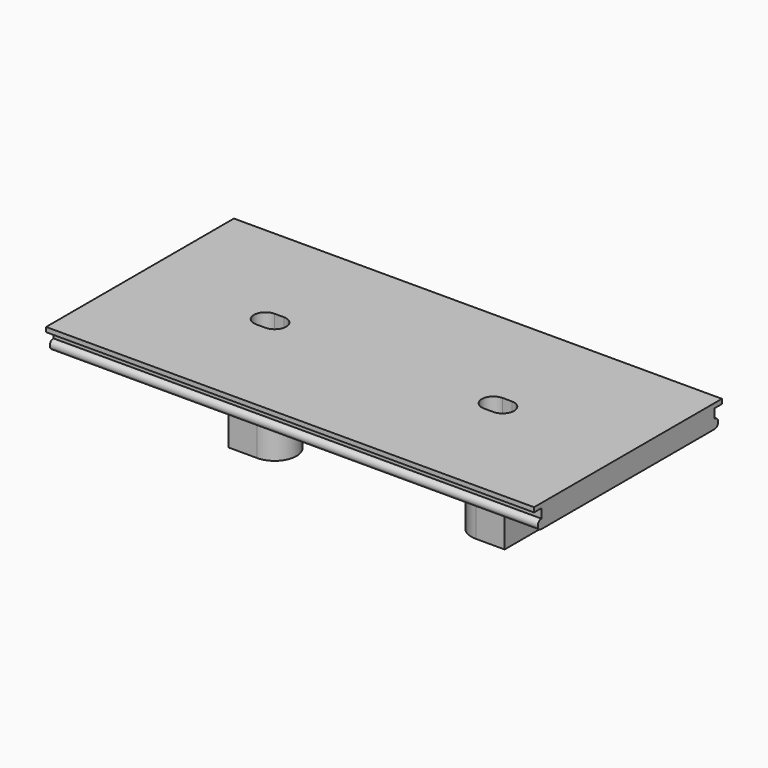
from build123d import *

# Parameters (mm, degrees)
F0_W     = 106
F0_H     = 47
F1_DEPTH = 2
F3_DEPTH = 1
F5_DEPTH = 106
F7_DEPTH = 19
F8_DEPTH = 25


with BuildPart() as f1:
    # F0 (on Top) → F1 (new body)
    with BuildSketch(Plane.XY):
        with Locations((53, 23.5)):
            Rectangle(F0_W, F0_H)
    extrude(amount=F1_DEPTH)

    # F2 (on face) → F3 (join)
    with BuildSketch(Plane.XY.offset(2)):
        Polygon((0, 49), (0, 0), (0, -2), (106, -2), (106, 49), align=None)
    extrude(amount=F3_DEPTH)

    # F4 (on face) → F5 (join)
    with BuildSketch(Plane.YZ.offset(106)):
        with BuildLine():
            Line((47, 0), (0, 0))
            ThreePointArc((0, 0), (-1, -1), (0, -2))
            Line((0, -2), (47, -2))
            ThreePointArc((47, -2), (48, -1), (47, 0))
        make_face()
    extrude(amount=-F5_DEPTH)

    # F6 (on face) → F7 (join)
    with BuildSketch(Plane(origin=(0, 0, -2), x_dir=(1, 0, 0), z_dir=(0, 0, -1))):
        with BuildLine():
            Line((23, -28.25), (29.25, -28.25))
            ThreePointArc((29.25, -28.25), (34, -23.5), (29.25, -18.75))
            Line((29.25, -18.75), (23, -18.75))
            Line((23, -18.75), (23, -28.25))
        make_face()
        with BuildLine():
            Line((27.25, -21), (29.25, -21))
            ThreePointArc((29.25, -21), (31.75, -23.5), (29.25, -26))
            Line((29.25, -26), (27.25, -26))
            ThreePointArc((27.25, -26), (24.75, -23.5), (27.25, -21))
        make_face(mode=Mode.SUBTRACT)
        with BuildLine():
            Line((83, -18.75), (76.75, -18.75))
            ThreePointArc((76.75, -18.75), (72, -23.5), (76.75, -28.25))
            Line((76.75, -28.25), (83, -28.25))
            Line((83, -28.25), (83, -18.75))
        make_face()
        with BuildLine():
            ThreePointArc((76.75, -26), (74.25, -23.5), (76.75, -21))
            Line((76.75, -21), (78.75, -21))
            ThreePointArc((78.75, -21), (81.25, -23.5), (78.75, -26))
            Line((78.75, -26), (76.75, -26))
        make_face(mode=Mode.SUBTRACT)
    extrude(amount=F7_DEPTH)

    # F8 (cut): faces of the model
    f8_faces = [f1.faces().sort_by_distance(p)[0] for p in [
        (28.25, 23.5, -2),
        (77.75, 23.5, -2),
    ]]
    extrude(f8_faces, amount=-F8_DEPTH, mode=Mode.SUBTRACT)


solid = f1.part
